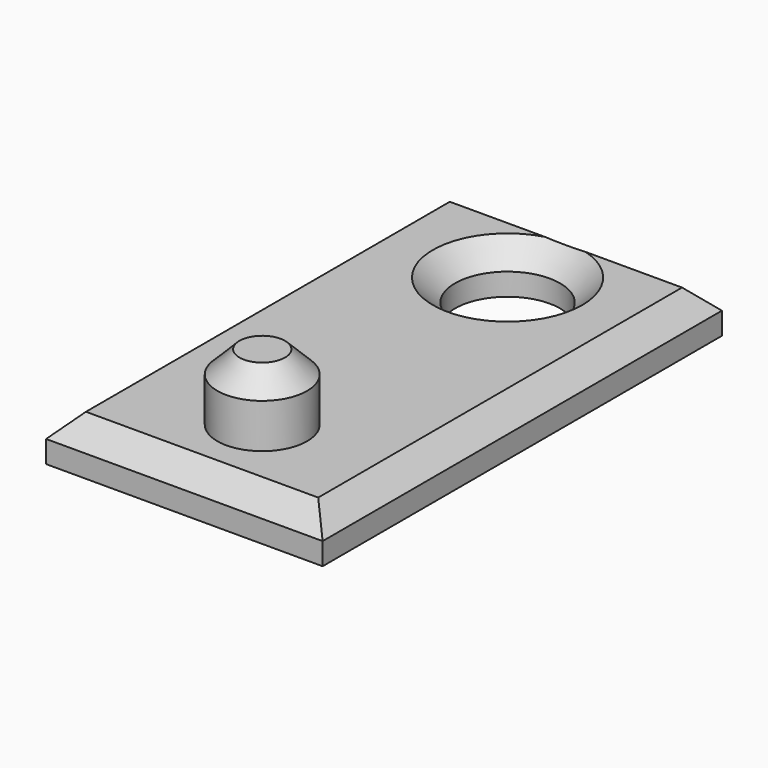
from build123d import *

# Parameters (mm, degrees)
F0_W         = 62.4540001154
F0_H         = 112.7128452063
F1_DEPTH     = 10
F3_R         = 11.8634694321
F4_DEPTH     = 25
F6_R         = 10.1380548027
F7_DEPTH     = 25
F9_SIZE      = 5
F10_T1_DEPTH = 133.4296750859
F10_T3_DEPTH = 88.1708299951


# Not quite as in the source:
# - a fillet or chamfer that OpenCascade refuses, or shapes differently, is made with other operations: its cross-section is extruded or revolved along the edge and cut away or added


with BuildPart() as f1:
    # F0 (on Top) → F1 (new body)
    with BuildSketch(Plane.XY):
        with Locations((31.2270000577, -6.0975924134)):
            Rectangle(F0_W, F0_H)
    extrude(amount=F1_DEPTH)

    # F3 (on face) → F4 (cut)
    with BuildSketch(Plane.XY.offset(10)):
        with Locations((31.0296863317, 29.0262252092)):
            Circle(F3_R)
    extrude(amount=-F4_DEPTH, mode=Mode.SUBTRACT)

    # F6 (on Top) → F7 (join)
    with BuildSketch(Plane.XY):
        with Locations((32.3501564562, -41.873395443)):
            Circle(F6_R)
    extrude(amount=F7_DEPTH)

    # F9
    f9_edges = [f1.edges().sort_by_distance(p)[0] for p in [
        (31.227, 50.25883, 10),
    ]]
    chamfer(f9_edges, length=F9_SIZE)

    # F10: chamfer of 5 on 5 edges, made by hand

    # F10_s2 → F10_t1 (cut)
    with BuildSketch(Plane.XZ.offset(-58.1172451295)):
        Polygon((57.4540001154, 10), (62.4540001154, 5), (62.4540001154, 10), align=None)
        Polygon((0, 5), (5, 10), (0, 10), align=None)
    extrude(amount=F10_T1_DEPTH, mode=Mode.SUBTRACT)

    # F10_s4 → F10_t3 (cut)
    with BuildSketch(Plane.YZ.offset(-12.8584149398)):
        Polygon((-57.4540150166, 10), (-62.4540150166, 5), (-62.4540150166, 10), align=None)
    extrude(amount=F10_T3_DEPTH, mode=Mode.SUBTRACT)

    # F10_s5 → F10_t6 (revolve, cut)
    with BuildSketch(Plane.XZ.offset(41.873395443)):
        Polygon((42.488211259, 20), (37.488211259, 25), (42.488211259, 25), align=None)
    revolve(axis=Axis((32.3501564562, -41.873395443, 25), (0, 0, 1)), mode=Mode.SUBTRACT)

    # F10_s7 → F10_t8 (revolve, cut)
    with BuildSketch(Plane.XZ.offset(-29.0262252092)):
        Polygon((47.8931557638, 10), (42.8931557638, 5), (42.8931557638, 10), align=None)
    revolve(axis=Axis((31.0296863317, 29.0262252092, 10), (0, 0, 1)), mode=Mode.SUBTRACT)


solid = f1.part
